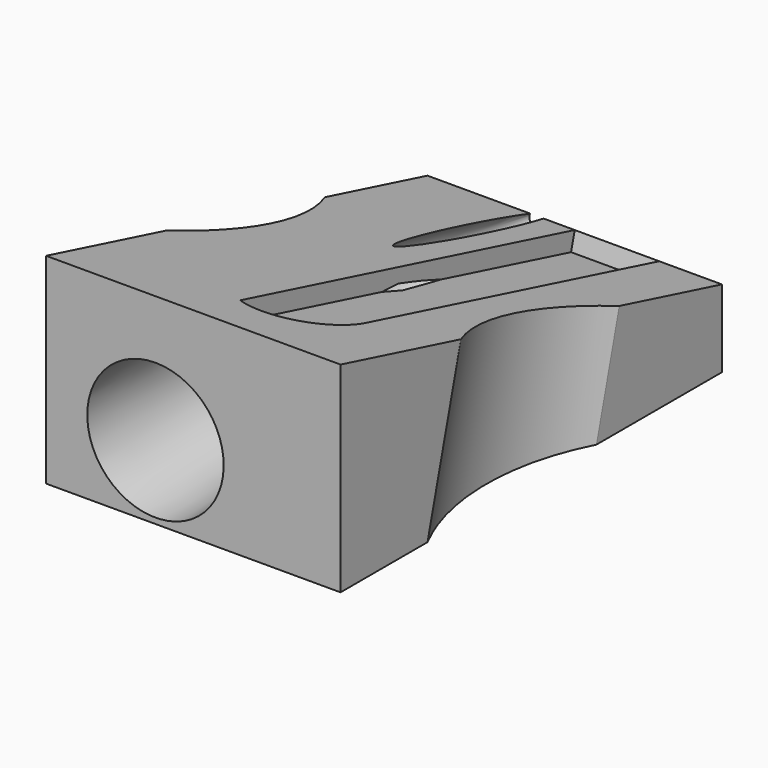
from build123d import *

# Parameters (mm, degrees)
F0_W      = 26.15
F0_H      = 11
F1_DEPTH  = 16.15
F3_DEPTH  = 25
F5_DEPTH  = 1
F13_DEPTH = 10


# Not quite as in the source:
# - the program builds the solid bodies; features that only make, move or delete a surface that nothing else refers to are left out


with BuildPart() as f1:
    # F0 (on Right) → F1 (new body)
    with BuildSketch(Plane.YZ):
        with Locations((6.6714687273, -5.5)):
            Rectangle(F0_W, F0_H)
    extrude(amount=F1_DEPTH)

    # F2 (on face) → F3 (cut)
    with BuildSketch(Plane(origin=(0, 0, 0), x_dir=(0, -1, 0), z_dir=(-1, 0, 0))):
        Polygon((-19.7464687273, -6.7590326071), (6.4035312727, 0), (-19.7464687273, 0), align=None)
    extrude(amount=-F3_DEPTH, mode=Mode.SUBTRACT)

    # F4 (on face) → F5 (cut)
    with BuildSketch(Plane(origin=(0, -0.4010136369, -1.5514803987), x_dir=(1, 0, 0), z_dir=(0, 0.2502475322, 0.9681818903))):
        with BuildLine():
            Line((12.7111524343, 0), (12.7111524343, 20.8096046483))
            Line((12.7111524343, 20.8096046483), (8.075, 20.8096046483))
            Line((8.075, 20.8096046483), (8.075, -2.8755263988))
            ThreePointArc((8.075, -2.8755263988), (11.1931797197, -2.7277537217), (12.7111524343, 0))
        make_face()
    extrude(amount=-F5_DEPTH, mode=Mode.SUBTRACT)

    # F9 (on offset) → F10 (revolve, cut)
    with BuildSketch(Plane.YZ.offset(6)):
        Polygon((7.6412414201, -3.6817420176), (-6.7182444036, -3.1987416248), (-6.7182444036, -6.9507951848), (7.6412414201, -6.9507951848), align=None)
        Polygon((19.8289547116, -6.5558860078), (7.6412414201, -3.6817420176), (7.6412414201, -6.9507951848), (19.8289547116, -6.9507951848), align=None)
    revolve(axis=Axis((6, 0.4614985082, -6.9507951848), (0, -1, 0)), mode=Mode.SUBTRACT)

    # F9 (on offset) → F11 (revolve, cut)
    with BuildSketch(Plane.YZ.offset(6)):
        Polygon((19.8289547116, -6.5558860078), (7.6412414201, -3.6817420176), (7.6412414201, -6.9507951848), (19.8289547116, -6.9507951848), align=None)
    revolve(axis=Axis((6, 13.7350980658, -6.9507951848), (0, 1, 0)), mode=Mode.SUBTRACT)

    # F12 (on face) → F13 (cut)
    with BuildSketch(Plane(origin=(0, -0.4010136369, -1.5514803987), x_dir=(1, 0, 0), z_dir=(0, 0.2502475322, 0.9681818903))):
        with BuildLine():
            Line((0, 13.5377381568), (0, 2.3293004092))
            ThreePointArc((0, 2.3293004092), (1.4062806348, 7.933519283), (0, 13.5377381568))
        make_face()
        with BuildLine():
            Line((16.15, 2.3293004092), (16.15, 13.5377381568))
            ThreePointArc((16.15, 13.5377381568), (14.7437193652, 7.933519283), (16.15, 2.3293004092))
        make_face()
    extrude(amount=-F13_DEPTH, mode=Mode.SUBTRACT)


solid = f1.part
